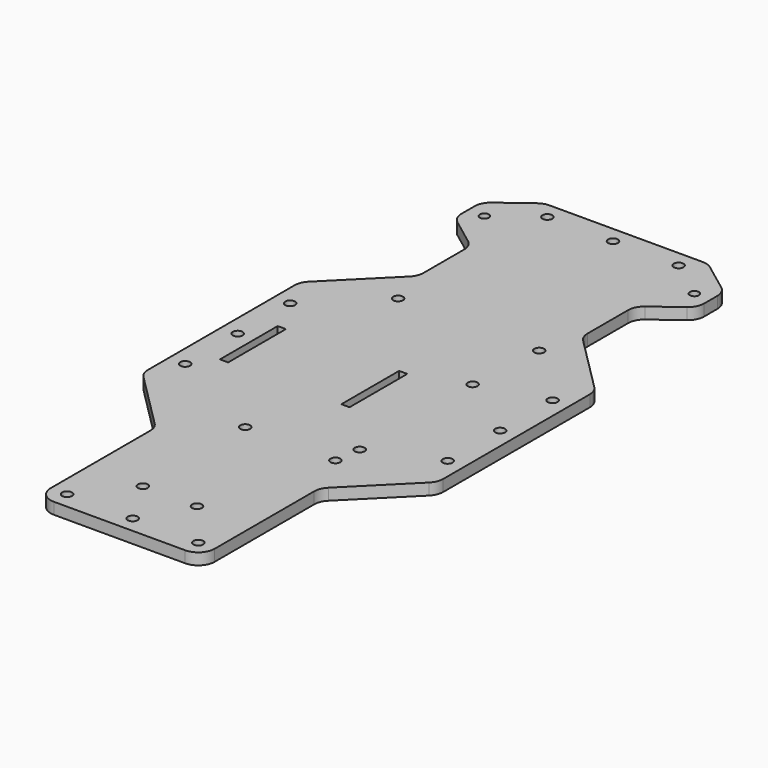
from build123d import *

# Parameters (mm, degrees)
F0_R     = 1.5
F0_W     = 2.5
F0_H     = 22
F0_R_2   = 1.375
F1_DEPTH = 3.5
F2_R     = 5


# Not quite as in the source:
# - a feature names something its author has since deleted; it is built from what else it names


with BuildPart() as f1:
    # F0 (on Top) → F1 (new body)
    with BuildSketch(Plane.XY):
        with BuildLine():
            Line((-25, 52), (-45, 32))
            Line((-45, 32), (-45, -28))
            Line((-45, -28), (-25, -48))
            Line((-25, -48), (-25, -88))
            ThreePointArc((-25, -88), (-23.5355339059, -91.5355339059), (-20, -93))
            Line((-20, -93), (20, -93))
            ThreePointArc((20, -93), (23.5355339059, -91.5355339059), (25, -88))
            Line((25, -88), (25, -48))
            Line((25, -48), (45, -28))
            Line((45, -28), (45, 32))
            Line((45, 32), (25, 52))
            Line((25, 52), (25, 72))
            Line((25, 72), (37, 81))
            Line((37, 81), (37, 91))
            Line((37, 91), (25, 100))
            Line((25, 100), (-25, 100))
            Line((-25, 100), (-37, 91))
            Line((-37, 91), (-37, 81))
            Line((-37, 81), (-25, 72))
            Line((-25, 72), (-25, 52))
        make_face()
        with Locations((-20, -88)):
            Circle(F0_R, mode=Mode.SUBTRACT)
        with Locations((-8.5, -73.5)):
            Circle(F0_R, mode=Mode.SUBTRACT)
        with Locations((-40, -18)):
            Circle(F0_R, mode=Mode.SUBTRACT)
        with Locations((-40, 2)):
            Circle(F0_R, mode=Mode.SUBTRACT)
        with Locations((-33.75, 0)):
            Rectangle(F0_W, F0_H, mode=Mode.SUBTRACT)
        with Locations((-8.5, -34.5)):
            Circle(F0_R, mode=Mode.SUBTRACT)
        with Locations((0, -88)):
            Circle(F0_R, mode=Mode.SUBTRACT)
        with Locations((8, -73.5)):
            Circle(F0_R, mode=Mode.SUBTRACT)
        with Locations((20, -88)):
            Circle(F0_R, mode=Mode.SUBTRACT)
        with Locations((19, -34.5)):
            Circle(F0_R, mode=Mode.SUBTRACT)
        with Locations((20, -26.5)):
            Circle(F0_R, mode=Mode.SUBTRACT)
        with Locations((3.25, 0)):
            Rectangle(F0_W, F0_H, mode=Mode.SUBTRACT)
        with Locations((40, -18)):
            Circle(F0_R, mode=Mode.SUBTRACT)
        with Locations((40, 2)):
            Circle(F0_R, mode=Mode.SUBTRACT)
        with Locations((-40, 22)):
            Circle(F0_R, mode=Mode.SUBTRACT)
        with Locations((-21.5, 40)):
            Circle(F0_R, mode=Mode.SUBTRACT)
        with Locations((-32, 86)):
            Circle(F0_R_2, mode=Mode.SUBTRACT)
        with Locations((-20, 95)):
            Circle(F0_R, mode=Mode.SUBTRACT)
        with Locations((20, 16.5)):
            Circle(F0_R, mode=Mode.SUBTRACT)
        with Locations((21.5, 40)):
            Circle(F0_R, mode=Mode.SUBTRACT)
        with Locations((40, 22)):
            Circle(F0_R, mode=Mode.SUBTRACT)
        with Locations((0, 95)):
            Circle(F0_R, mode=Mode.SUBTRACT)
        with Locations((20, 95)):
            Circle(F0_R, mode=Mode.SUBTRACT)
        with Locations((32, 86)):
            Circle(F0_R_2, mode=Mode.SUBTRACT)
    extrude(amount=F1_DEPTH)

    # F2
    f2_edges = [f1.edges().sort_by_distance(p)[0] for p in [
        (-45, -28, 1.75),
        (-25, -48, 1.75),
        (25, -48, 1.75),
        (45, -28, 1.75),
        (45, 32, 1.75),
        (25, 52, 1.75),
        (25, 72, 1.75),
        (-25, 52, 1.75),
        (-45, 32, 1.75),
        (-25, 72, 1.75),
        (-37, 81, 1.75),
        (-37, 91, 1.75),
        (-25, 100, 1.75),
        (25, 100, 1.75),
        (37, 91, 1.75),
        (37, 81, 1.75),
    ]]
    fillet(f2_edges, radius=F2_R)


solid = f1.part
